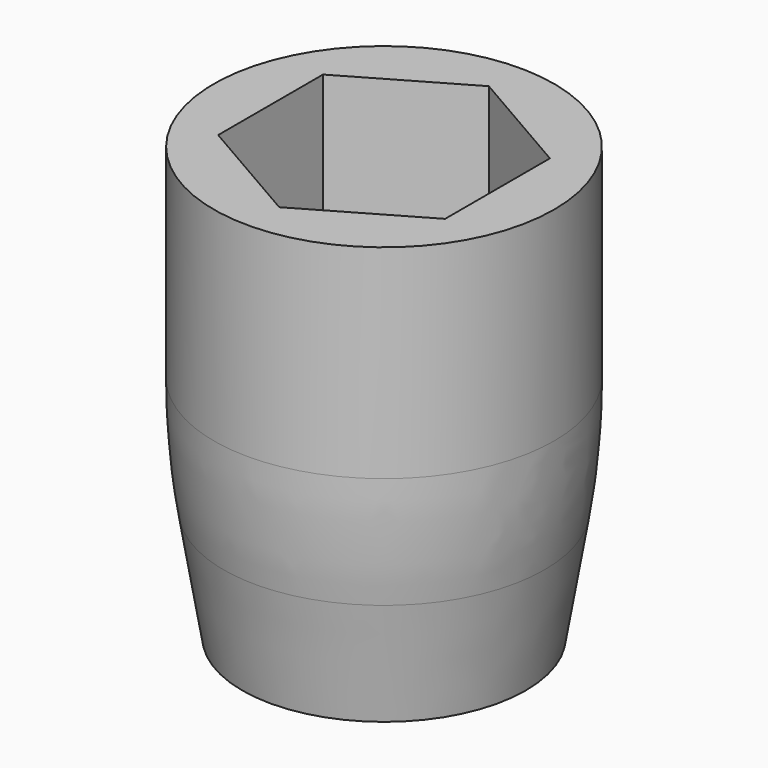
from build123d import *

# Parameters (mm, degrees)
F0_R     = 12
F1_DEPTH = 18.5
F0_W     = 10.1
F0_H     = 10.1
F2_DEPTH = 12
F3_SIZE2 = 11.99999
F3_SIZE  = 1.99999
F4_R     = 1
F5_R     = 0.7
F6_R     = 50
F7_SIZE  = 0.8


# Not quite as in the source:
# - a fillet or chamfer is up to 0.001 mm smaller than in the source, because OpenCascade refuses the exact size


with BuildPart() as f1:
    # F0 (on Top) → F1 (new body)
    with BuildSketch(Plane.XY):
        Circle(F0_R)
        Polygon((0, 9.237604307), (8, 4.6188021535), (8, -4.6188021535), (0, -9.237604307), (-8, -4.6188021535), (-8, 4.6188021535), align=None, mode=Mode.SUBTRACT)
    extrude(amount=F1_DEPTH)

    # F0 (on Top) → F2 (join)
    with BuildSketch(Plane.XY):
        Circle(F0_R)
        Polygon((0, 9.237604307), (8, 4.6188021535), (8, -4.6188021535), (0, -9.237604307), (-8, -4.6188021535), (-8, 4.6188021535), align=None, mode=Mode.SUBTRACT)
        Polygon((8, -4.6188021535), (8, 4.6188021535), (0, 9.237604307), (-8, 4.6188021535), (-8, -4.6188021535), (0, -9.237604307), align=None)
        Rectangle(F0_W, F0_H, mode=Mode.SUBTRACT)
    extrude(amount=-F2_DEPTH)

    # F3 (size 2 and 12 in the source; OpenCascade refuses exactly that, so slightly less here)
    f3_edges = [f1.edges().sort_by_distance(p)[0] for p in [
        (-12, 0, -12),
    ]]
    f3_side = f1.faces().sort_by_distance((5.389411, 0, -12))[0]
    chamfer(f3_edges, length=F3_SIZE, length2=F3_SIZE2, reference=f3_side)

    # F4
    f4_edges = [f1.edges().sort_by_distance(p)[0] for p in [
        (-5.05, 5.05, -6),
        (5.05, 5.05, -6),
        (5.05, -5.05, -6),
        (-5.05, -5.05, -6),
    ]]
    fillet(f4_edges, radius=F4_R)

    # F5
    f5_edges = [f1.edges().sort_by_distance(p)[0] for p in [
        (4, -6.928203, 0),
        (-4, -6.928203, 0),
        (5.05, 0, 0),
        (4.757107, 4.757107, 0),
        (4.757107, -4.757107, 0),
        (0, 5.05, 0),
        (0, -5.05, 0),
        (-4.757107, 4.757107, 0),
        (-4.757107, -4.757107, 0),
        (-5.05, 0, 0),
        (-4, 6.928203, 0),
        (4, 6.928203, 0),
        (8, 0, 0),
        (-8, 0, 0),
    ]]
    fillet(f5_edges, radius=F5_R)

    # F6
    f6_edges = [f1.edges().sort_by_distance(p)[0] for p in [
        (-12, 0, -1e-05),
        (-12, 0, 0),
    ]]
    fillet(f6_edges, radius=F6_R)

    # F7
    f7_edges = [f1.edges().sort_by_distance(p)[0] for p in [
        (5.05, 0, -12),
    ]]
    chamfer(f7_edges, length=F7_SIZE)


solid = f1.part
